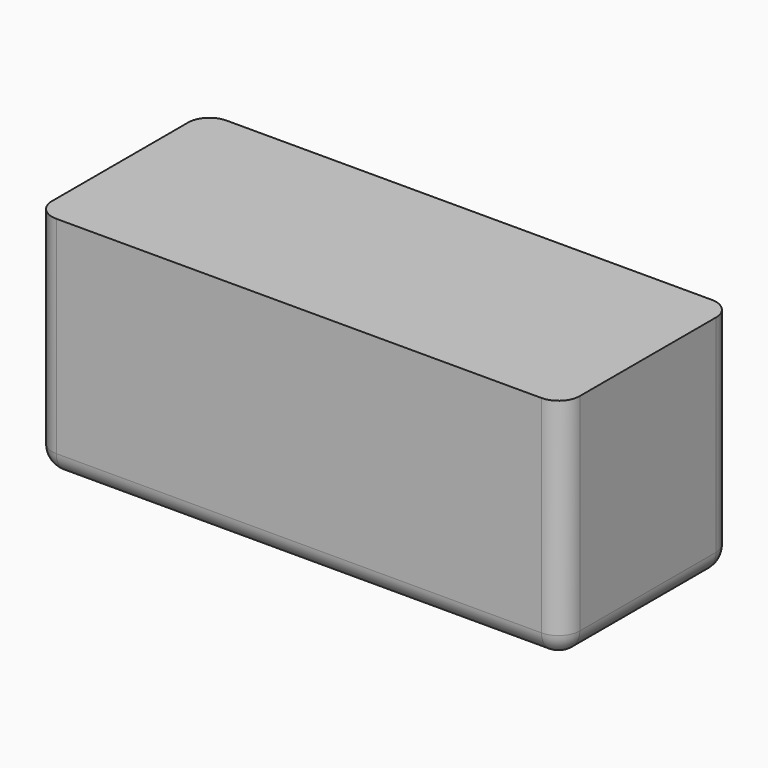
from build123d import *

# Parameters (mm, degrees)
F0_W         = 126.0307952762
F0_H         = 54.4428955764
F1_DEPTH     = 50.8
F2_R         = 5.08
F3_T1_DEPTH  = 62.0628955764
F3_S5_W      = 5.08
F3_S5_H      = 5.08
F3_T6_DEPTH  = 5.08
F3_S11_W     = 5.08
F3_S11_H     = 5.08
F3_T12_DEPTH = 5.08
F4_DEPTH     = 47.752


# Not quite as in the source:
# - a fillet or chamfer that OpenCascade refuses, or shapes differently, is made with other operations: its cross-section is extruded or revolved along the edge and cut away or added


with BuildPart() as f1:
    # F0 (on Front) → F1 (new body)
    with BuildSketch(Plane.XZ):
        with Locations((3.3086873591, 6.0157896951)):
            Rectangle(F0_W, F0_H)
    extrude(amount=F1_DEPTH)

    # F2
    f2_edges = [f1.edges().sort_by_distance(p)[0] for p in [
        (66.324085, -50.8, 6.01579),
        (-59.70671, -50.8, 6.01579),
        (3.308687, -50.8, -21.205658),
        (-59.70671, -25.4, -21.205658),
        (66.324085, -25.4, -21.205658),
        (3.308687, 0, -21.205658),
    ]]
    fillet(f2_edges, radius=F2_R)

    # F3: fillet of radius 5.08 on 2 edges, made by hand

    # F3_s2 → F3_t1 (cut)
    with BuildSketch(Plane.XY.offset(-16.1256580931)):
        with BuildLine():
            ThreePointArc((66.3240849972, -5.08), (64.8361874456, -1.4878975516), (61.2440849972, 0))
            Line((61.2440849972, 0), (66.3240849972, 0))
            Line((66.3240849972, 0), (66.3240849972, -5.08))
        make_face()
        with BuildLine():
            ThreePointArc((-54.626710279, 0), (-58.2188127274, -1.4878975516), (-59.706710279, -5.08))
            Line((-59.706710279, -5.08), (-59.706710279, 0))
            Line((-59.706710279, 0), (-54.626710279, 0))
        make_face()
    extrude(amount=F3_T1_DEPTH, mode=Mode.SUBTRACT)


with BuildPart() as f3_tool4:
    # F3_s5 → F3_t6 (new body)
    with BuildSketch(Plane.XZ.offset(5.08)):
        with Locations((-57.166710279, -18.6656580931)):
            Rectangle(F3_S5_W, F3_S5_H)
    extrude(amount=-F3_T6_DEPTH)

    # F3_s7 → F3_t8 (revolve, cut)
    with BuildSketch(Plane(origin=(-54.626710279, -5.08, -16.1256580931), x_dir=(0.7071067812, 0, 0.7071067812), z_dir=(-0.7071067812, 0, 0.7071067812))):
        with BuildLine():
            ThreePointArc((0, -5.08), (5.08, 0), (0, 5.08))
            Line((0, 5.08), (0, -5.08))
        make_face()
    revolve(axis=Axis((-54.626710279, -5.08, -16.1256580931), (0, 1, 0)), mode=Mode.SUBTRACT)


with BuildPart() as f1_1:
    add(f1.part)

    # F3_t3: cut F3_tool4
    add(f3_tool4.part, mode=Mode.SUBTRACT)


with BuildPart() as f3_tool10:
    # F3_s11 → F3_t12 (new body)
    with BuildSketch(Plane.YZ.offset(61.2440849972)):
        with Locations((-2.54, -18.6656580931)):
            Rectangle(F3_S11_W, F3_S11_H)
    extrude(amount=F3_T12_DEPTH)

    # F3_s13 → F3_t14 (revolve, cut)
    with BuildSketch(Plane(origin=(61.2440849972, -5.08, -16.1256580931), x_dir=(0, -0.7071067812, 0.7071067812), z_dir=(0, 0.7071067812, 0.7071067812))):
        with BuildLine():
            ThreePointArc((0, -5.08), (5.08, 0), (0, 5.08))
            Line((0, 5.08), (0, -5.08))
        make_face()
    revolve(axis=Axis((61.2440849972, -5.08, -16.1256580931), (1, 0, 0)), mode=Mode.SUBTRACT)


with BuildPart() as f1_2:
    add(f1_1.part)

    # F3_t9: cut F3_tool10
    add(f3_tool10.part, mode=Mode.SUBTRACT)

    # F4 (cut): a face of the model
    f4_faces = [f1_2.faces().sort_by_distance(p)[0] for p in [
        (3.3086873591, -25.4, -21.2056580931),
    ]]
    extrude(f4_faces, amount=-F4_DEPTH, mode=Mode.SUBTRACT)


solid = f1_2.part
